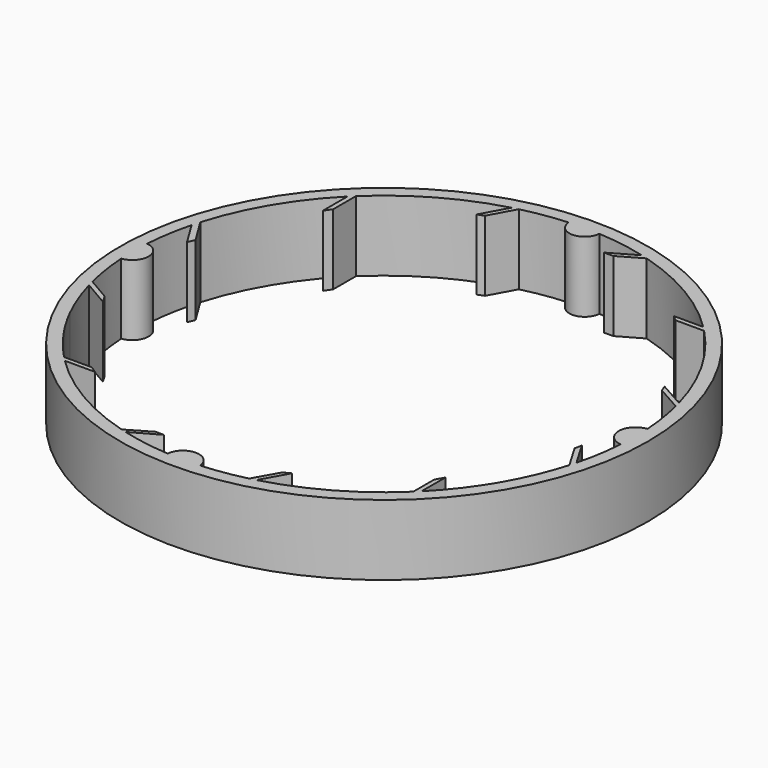
from build123d import *

# Parameters (mm, degrees)
F0_R     = 37.4226300925
F1_DEPTH = 10


with BuildPart() as f1:
    # F0 (on Top) → F1 (new body)
    with BuildSketch(Plane.XY):
        Circle(F0_R)
        with BuildLine():
            ThreePointArc((-8.5269049855, 34.5365748806), (-5.4052755249, 35.1605760706), (-2.2403607921, 35.5030125009))
            ThreePointArc((-2.2403607921, 35.5030125009), (-0.0668734001, 35.5735666059), (2.1068638934, 35.5111846839))
            ThreePointArc((2.1068638934, 35.5111846839), (5.5820572148, 35.1329439468), (9.0033478551, 34.4154447962))
            Line((9.0033478551, 34.4154447962), (5.3277746774, 32.3108322918))
            Line((5.3277746774, 32.3108322918), (6.6450131126, 32.3108322918))
            Line((6.6450131126, 32.3108322918), (9.8926773092, 34.1704265231))
            ThreePointArc((9.8926773092, 34.1704265231), (18.0341344438, 30.6635468917), (25.0557426886, 25.2525814807))
            Line((25.0557426886, 25.2525814807), (20.8670180282, 25.2525814807))
            Line((20.8670180282, 25.2525814807), (21.6717198491, 24.5820395648))
            Line((21.6717198491, 24.5820395648), (25.7139348204, 24.5820395648))
            ThreePointArc((25.7139348204, 24.5820395648), (30.970985058, 17.5008913388), (34.3244938146, 9.3441017486))
            Line((34.3244938146, 9.3441017486), (30.6226182729, 11.4265037701))
            Line((30.6226182729, 11.4265037701), (30.9700332582, 10.5129266158))
            Line((30.9700332582, 10.5129266158), (34.5408713256, 8.5094841905))
            ThreePointArc((34.5408713256, 8.5094841905), (35.1576024678, 5.4245831021), (35.4993763194, 2.2972579413))
            ThreePointArc((35.4993763194, 2.2972579413), (33.326526558, -0.0646682307), (35.4901936241, -2.4350091671))
            ThreePointArc((35.4901936241, -2.4350091671), (35.1114069781, -5.7159612611), (34.4299693949, -8.9476432978))
            Line((34.4299693949, -8.9476432978), (32.3091186583, -5.346425809))
            Line((32.3091186583, -5.346425809), (32.1022830904, -6.364681758))
            Line((32.1022830904, -6.364681758), (34.1735842261, -9.8817637222))
            ThreePointArc((34.1735842261, -9.8817637222), (33.1529686946, -12.898208397), (31.8666911327, -15.8112968908))
            ThreePointArc((31.8666911327, -15.8112968908), (30.841049084, -17.7288692397), (29.700156108, -19.5801899959))
            ThreePointArc((29.700156108, -19.5801899959), (27.6349933602, -22.4006753268), (25.3029755485, -25.0048503597))
            Line((25.3029755485, -25.0048503597), (25.3181142434, -20.7694043622))
            Line((25.3181142434, -20.7694043622), (24.6594950259, -21.9101663099))
            Line((24.6594950259, -21.9101663099), (24.6461187726, -25.6525231228))
            ThreePointArc((24.6461187726, -25.6525231228), (17.5414682427, -30.9480210192), (9.3484371144, -34.3233133108))
            Line((9.3484371144, -34.3233133108), (11.4183174446, -30.5898860097))
            Line((11.4183174446, -30.5898860097), (10.4497633874, -31.0920979828))
            Line((10.4497633874, -31.0920979828), (8.4997417198, -34.543270022))
            ThreePointArc((8.4997417198, -34.543270022), (5.4306890655, -35.1566598156), (2.3196007667, -35.4979233956))
            ThreePointArc((2.3196007667, -35.4979233956), (0.0172965119, -33.3822489231), (-2.2828140972, -35.5003080679))
            ThreePointArc((-2.2828140972, -35.5003080679), (-5.7550130369, -35.1050272477), (-9.1716738253, -34.3709690343))
            Line((-9.1716738253, -34.3709690343), (-5.4097990505, -32.2477370501))
            Line((-5.4097990505, -32.2477370501), (-6.5905414522, -32.2477370501))
            Line((-6.5905414522, -32.2477370501), (-9.885855651, -34.1724007229))
            ThreePointArc((-9.885855651, -34.1724007229), (-18.0434280361, -30.6580791607), (-25.0760843465, -25.2323821104))
            Line((-25.0760843465, -25.2323821104), (-20.8179873924, -25.2323821104))
            Line((-20.8179873924, -25.2323821104), (-21.7606406659, -24.5914589614))
            Line((-21.7606406659, -24.5914589614), (-25.7049267509, -24.5914589614))
            ThreePointArc((-25.7049267509, -24.5914589614), (-27.7738883496, -22.2282306777), (-29.6263303406, -19.6917156101))
            ThreePointArc((-29.6263303406, -19.6917156101), (-30.7741756839, -17.8446973663), (-31.8070200014, -15.930994688))
            ThreePointArc((-31.8070200014, -15.930994688), (-33.2170505751, -12.73226862), (-34.3063234036, -9.4105944365))
            Line((-34.3063234036, -9.4105944365), (-30.6458889209, -11.5414279296))
            Line((-30.6458889209, -11.5414279296), (-31.3045081384, -10.400665982))
            Line((-31.3045081384, -10.400665982), (-34.5387960818, -8.5179034004))
            ThreePointArc((-34.5387960818, -8.5179034004), (-35.1643257366, -5.3808278739), (-35.505521273, -2.20024368))
            ThreePointArc((-35.505521273, -2.20024368), (-33.4584605706, 0.0814176869), (-35.4943927242, 2.3730145927))
            ThreePointArc((-35.4943927242, 2.3730145927), (-35.1180774116, 5.6748349785), (-34.435293299, 8.9271321558))
            Line((-34.435293299, 8.9271321558), (-32.2886370122, 5.4360465147))
            Line((-32.2886370122, 5.4360465147), (-31.8586565554, 6.4034969546))
            Line((-31.8586565554, 6.4034969546), (-34.1168341585, 10.0759485966))
            ThreePointArc((-34.1168341585, 10.0759485966), (-30.6126401352, 18.1204132699), (-25.2459538538, 25.0624206159))
            Line((-25.2459538538, 25.0624206159), (-25.2459538538, 20.6894481147))
            Line((-25.2459538538, 20.6894481147), (-24.5687514544, 21.6902010143))
            Line((-24.5687514544, 21.6902010143), (-24.5687514544, 25.7266314369))
            ThreePointArc((-24.5687514544, 25.7266314369), (-17.5076688048, 30.9671543113), (-9.3768544488, 34.3155608109))
            Line((-9.3768544488, 34.3155608109), (-11.3971997052, 30.6179970503))
            Line((-11.3971997052, 30.6179970503), (-10.4683693498, 30.9792086482))
            Line((-10.4683693498, 30.9792086482), (-8.5269049855, 34.5365748806))
        make_face(mode=Mode.SUBTRACT)
        with BuildLine():
            ThreePointArc((2.1068638934, 35.5111846839), (-0.0668734001, 35.5735666059), (-2.2403607921, 35.5030125009))
            ThreePointArc((-2.2403607921, 35.5030125009), (-0.0629027102, 33.4613425852), (2.1068638934, 35.5111846839))
        make_face()
    extrude(amount=F1_DEPTH)


solid = f1.part
